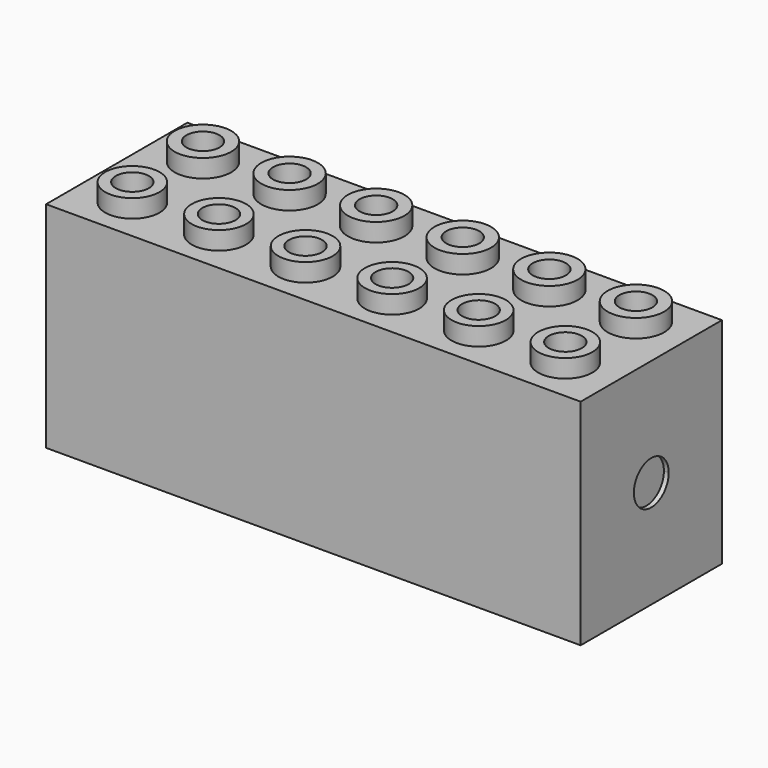
from build123d import *

# Parameters (mm, degrees)
F1_DEPTH  = 19.2532
F4_DEPTH  = 1.6256
F7_DEPTH  = 0.4318
F9_DEPTH  = 19.2532
F10_DEPTH = 2.032


with BuildPart() as f1:
    # F0 (on Top) → F1 (new body)
    with BuildSketch(Plane.XY):
        Polygon((0, 7.9248), (0, 0), (47.9806, 0), (47.9806, 7.9248), (46.4566, 7.9248), (46.4566, 1.524), (1.524, 1.524), (1.524, 7.9248), align=None)
        Polygon((0, 15.8496), (0, 7.9248), (1.524, 7.9248), (1.524, 14.3256), (46.4566, 14.3256), (46.4566, 7.9248), (47.9806, 7.9248), (47.9806, 15.8496), align=None)
    extrude(amount=F1_DEPTH)



with BuildPart() as f1b:
    # F0 (on Top) → F1, piece 2 (new body)
    with BuildSketch(Plane.XY):
        with BuildLine():
            ThreePointArc((36.6014, 7.9248), (39.8399, 4.6863), (43.0784, 7.9248))
            Line((43.0784, 7.9248), (42.2148, 7.9248))
            ThreePointArc((42.2148, 7.9248), (39.8399, 5.5499), (37.465, 7.9248))
            Line((37.465, 7.9248), (36.6014, 7.9248))
        make_face()
        with BuildLine():
            Line((42.2148, 7.9248), (43.0784, 7.9248))
            ThreePointArc((43.0784, 7.9248), (39.8399, 11.1633), (36.6014, 7.9248))
            Line((36.6014, 7.9248), (37.465, 7.9248))
            ThreePointArc((37.465, 7.9248), (39.8399, 10.2997), (42.2148, 7.9248))
        make_face()
    extrude(amount=F1_DEPTH)


with BuildPart() as f4:
    # F3 (on face) → F4 (new body)
    with BuildSketch(Plane.XY.offset(19.2532)):
        with BuildLine():
            ThreePointArc((7.0104, 3.9624), (4.572, 6.4008), (2.1336, 3.9624))
            Line((2.1336, 3.9624), (3.0861, 3.9624))
            ThreePointArc((3.0861, 3.9624), (4.572, 5.4483), (6.0579, 3.9624))
            Line((6.0579, 3.9624), (7.0104, 3.9624))
        make_face()
        with BuildLine():
            Line((3.0861, 3.9624), (2.1336, 3.9624))
            ThreePointArc((2.1336, 3.9624), (4.572, 1.524), (7.0104, 3.9624))
            Line((7.0104, 3.9624), (6.0579, 3.9624))
            ThreePointArc((6.0579, 3.9624), (4.572, 2.4765), (3.0861, 3.9624))
        make_face()
    extrude(amount=F4_DEPTH)


with BuildPart() as f4b:
    # F3 (on face) → F4, piece 2 (new body)
    with BuildSketch(Plane.XY.offset(19.2532)):
        with BuildLine():
            ThreePointArc((17.6784, 3.9624), (20.1168, 1.524), (22.5552, 3.9624))
            Line((22.5552, 3.9624), (21.6027, 3.9624))
            ThreePointArc((21.6027, 3.9624), (20.1168, 2.4765), (18.6309, 3.9624))
            Line((18.6309, 3.9624), (17.6784, 3.9624))
        make_face()
        with BuildLine():
            Line((21.6027, 3.9624), (22.5552, 3.9624))
            ThreePointArc((22.5552, 3.9624), (20.1168, 6.4008), (17.6784, 3.9624))
            Line((17.6784, 3.9624), (18.6309, 3.9624))
            ThreePointArc((18.6309, 3.9624), (20.1168, 5.4483), (21.6027, 3.9624))
        make_face()
    extrude(amount=F4_DEPTH)


with BuildPart() as f4c:
    # F3 (on face) → F4, piece 3 (new body)
    with BuildSketch(Plane.XY.offset(19.2532)):
        with BuildLine():
            ThreePointArc((30.3276, 3.9624), (27.8892, 6.4008), (25.4508, 3.9624))
            Line((25.4508, 3.9624), (26.4033, 3.9624))
            ThreePointArc((26.4033, 3.9624), (27.8892, 5.4483), (29.3751, 3.9624))
            Line((29.3751, 3.9624), (30.3276, 3.9624))
        make_face()
        with BuildLine():
            Line((26.4033, 3.9624), (25.4508, 3.9624))
            ThreePointArc((25.4508, 3.9624), (27.8892, 1.524), (30.3276, 3.9624))
            Line((30.3276, 3.9624), (29.3751, 3.9624))
            ThreePointArc((29.3751, 3.9624), (27.8892, 2.4765), (26.4033, 3.9624))
        make_face()
    extrude(amount=F4_DEPTH)


with BuildPart() as f4d:
    # F3 (on face) → F4, piece 4 (new body)
    with BuildSketch(Plane.XY.offset(19.2532)):
        with BuildLine():
            ThreePointArc((40.9956, 3.9624), (43.434, 1.524), (45.8724, 3.9624))
            Line((45.8724, 3.9624), (44.9199, 3.9624))
            ThreePointArc((44.9199, 3.9624), (43.434, 2.4765), (41.9481, 3.9624))
            Line((41.9481, 3.9624), (40.9956, 3.9624))
        make_face()
        with BuildLine():
            Line((44.9199, 3.9624), (45.8724, 3.9624))
            ThreePointArc((45.8724, 3.9624), (43.434, 6.4008), (40.9956, 3.9624))
            Line((40.9956, 3.9624), (41.9481, 3.9624))
            ThreePointArc((41.9481, 3.9624), (43.434, 5.4483), (44.9199, 3.9624))
        make_face()
    extrude(amount=F4_DEPTH)


with BuildPart() as f4e:
    # F3 (on face) → F4, piece 5 (new body)
    with BuildSketch(Plane.XY.offset(19.2532)):
        with BuildLine():
            ThreePointArc((14.7828, 3.9624), (12.3444, 6.4008), (9.906, 3.9624))
            Line((9.906, 3.9624), (10.8585, 3.9624))
            ThreePointArc((10.8585, 3.9624), (12.3444, 5.4483), (13.8303, 3.9624))
            Line((13.8303, 3.9624), (14.7828, 3.9624))
        make_face()
        with BuildLine():
            Line((10.8585, 3.9624), (9.906, 3.9624))
            ThreePointArc((9.906, 3.9624), (12.3444, 1.524), (14.7828, 3.9624))
            Line((14.7828, 3.9624), (13.8303, 3.9624))
            ThreePointArc((13.8303, 3.9624), (12.3444, 2.4765), (10.8585, 3.9624))
        make_face()
    extrude(amount=F4_DEPTH)


with BuildPart() as f4f:
    # F3 (on face) → F4, piece 6 (new body)
    with BuildSketch(Plane.XY.offset(19.2532)):
        with BuildLine():
            ThreePointArc((38.1, 3.9624), (35.6616, 6.4008), (33.2232, 3.9624))
            Line((33.2232, 3.9624), (34.1757, 3.9624))
            ThreePointArc((34.1757, 3.9624), (35.6616, 5.4483), (37.1475, 3.9624))
            Line((37.1475, 3.9624), (38.1, 3.9624))
        make_face()
        with BuildLine():
            Line((34.1757, 3.9624), (33.2232, 3.9624))
            ThreePointArc((33.2232, 3.9624), (35.6616, 1.524), (38.1, 3.9624))
            Line((38.1, 3.9624), (37.1475, 3.9624))
            ThreePointArc((37.1475, 3.9624), (35.6616, 2.4765), (34.1757, 3.9624))
        make_face()
    extrude(amount=F4_DEPTH)


with BuildPart() as f1_1:
    add(f1.part)

    add(f1b.part)  # F4#7 merges F1b
    # F3 (on face) → F4, piece 7 (join)
    with BuildSketch(Plane.XY.offset(19.2532)):
        with BuildLine():
            ThreePointArc((7.1105154008, 11.8872), (4.572, 14.4257154008), (2.0334845992, 11.8872))
            Line((2.0334845992, 11.8872), (3.0861, 11.8872))
            ThreePointArc((3.0861, 11.8872), (4.572, 13.3731), (6.0579, 11.8872))
            Line((6.0579, 11.8872), (7.1105154008, 11.8872))
        make_face()
        with BuildLine():
            Line((3.0861, 11.8872), (2.0334845992, 11.8872))
            ThreePointArc((2.0334845992, 11.8872), (4.572, 9.3486845992), (7.1105154008, 11.8872))
            Line((7.1105154008, 11.8872), (6.0579, 11.8872))
            ThreePointArc((6.0579, 11.8872), (4.572, 10.4013), (3.0861, 11.8872))
        make_face()
        with BuildLine():
            ThreePointArc((40.8954845992, 11.8872), (43.434, 9.3486845992), (45.9725154008, 11.8872))
            Line((45.9725154008, 11.8872), (44.9199, 11.8872))
            ThreePointArc((44.9199, 11.8872), (43.434, 10.4013), (41.9481, 11.8872))
            Line((41.9481, 11.8872), (40.8954845992, 11.8872))
        make_face()
        with BuildLine():
            Line((44.9199, 11.8872), (45.9725154008, 11.8872))
            ThreePointArc((45.9725154008, 11.8872), (43.434, 14.4257154008), (40.8954845992, 11.8872))
            Line((40.8954845992, 11.8872), (41.9481, 11.8872))
            ThreePointArc((41.9481, 11.8872), (43.434, 13.3731), (44.9199, 11.8872))
        make_face()
        with BuildLine():
            ThreePointArc((14.8829154008, 11.8872), (12.3444, 14.4257154008), (9.8058845992, 11.8872))
            Line((9.8058845992, 11.8872), (10.8585, 11.8872))
            ThreePointArc((10.8585, 11.8872), (12.3444, 13.3731), (13.8303, 11.8872))
            Line((13.8303, 11.8872), (14.8829154008, 11.8872))
        make_face()
        with BuildLine():
            Line((10.8585, 11.8872), (9.8058845992, 11.8872))
            ThreePointArc((9.8058845992, 11.8872), (12.3444, 9.3486845992), (14.8829154008, 11.8872))
            Line((14.8829154008, 11.8872), (13.8303, 11.8872))
            ThreePointArc((13.8303, 11.8872), (12.3444, 10.4013), (10.8585, 11.8872))
        make_face()
        with BuildLine():
            ThreePointArc((33.1230845992, 11.8872), (35.6616, 9.3486845992), (38.2001154008, 11.8872))
            Line((38.2001154008, 11.8872), (37.1475, 11.8872))
            ThreePointArc((37.1475, 11.8872), (35.6616, 10.4013), (34.1757, 11.8872))
            Line((34.1757, 11.8872), (33.1230845992, 11.8872))
        make_face()
        with BuildLine():
            Line((37.1475, 11.8872), (38.2001154008, 11.8872))
            ThreePointArc((38.2001154008, 11.8872), (35.6616, 14.4257154008), (33.1230845992, 11.8872))
            Line((33.1230845992, 11.8872), (34.1757, 11.8872))
            ThreePointArc((34.1757, 11.8872), (35.6616, 13.3731), (37.1475, 11.8872))
        make_face()
        with BuildLine():
            ThreePointArc((22.6553154008, 11.8872), (20.1168, 14.4257154008), (17.5782845992, 11.8872))
            Line((17.5782845992, 11.8872), (18.6309, 11.8872))
            ThreePointArc((18.6309, 11.8872), (20.1168, 13.3731), (21.6027, 11.8872))
            Line((21.6027, 11.8872), (22.6553154008, 11.8872))
        make_face()
        with BuildLine():
            Line((18.6309, 11.8872), (17.5782845992, 11.8872))
            ThreePointArc((17.5782845992, 11.8872), (20.1168, 9.3486845992), (22.6553154008, 11.8872))
            Line((22.6553154008, 11.8872), (21.6027, 11.8872))
            ThreePointArc((21.6027, 11.8872), (20.1168, 10.4013), (18.6309, 11.8872))
        make_face()
        with BuildLine():
            ThreePointArc((25.3506845992, 11.8872), (27.8892, 9.3486845992), (30.4277154008, 11.8872))
            Line((30.4277154008, 11.8872), (29.3751, 11.8872))
            ThreePointArc((29.3751, 11.8872), (27.8892, 10.4013), (26.4033, 11.8872))
            Line((26.4033, 11.8872), (25.3506845992, 11.8872))
        make_face()
        with BuildLine():
            Line((29.3751, 11.8872), (30.4277154008, 11.8872))
            ThreePointArc((30.4277154008, 11.8872), (27.8892, 14.4257154008), (25.3506845992, 11.8872))
            Line((25.3506845992, 11.8872), (26.4033, 11.8872))
            ThreePointArc((26.4033, 11.8872), (27.8892, 13.3731), (29.3751, 11.8872))
        make_face()
    extrude(amount=F4_DEPTH)

    # F6 (on offset) → F7 (cut)
    with BuildSketch(Plane.YZ.offset(47.9806)):
        with BuildLine():
            ThreePointArc((9.1678369266, 11.1365711385), (6.4148288615, 10.8696369266), (6.6817630734, 8.1166288615))
            Line((6.6817630734, 8.1166288615), (9.1678369266, 11.1365711385))
        make_face()
        with BuildLine():
            Line((9.1678369266, 11.1365711385), (6.6817630734, 8.1166288615))
            ThreePointArc((6.6817630734, 8.1166288615), (8.7596718521, 7.8579444002), (9.8806, 9.6266))
            ThreePointArc((9.8806, 9.6266), (9.6934555998, 10.4614718521), (9.1678369266, 11.1365711385))
        make_face()
    extrude(amount=-F7_DEPTH, mode=Mode.SUBTRACT)

    # F0 (on Top) → F9 (join)
    with BuildSketch(Plane.XY):
        with BuildLine():
            Line((4.9022, 7.9248), (1.524, 7.9248))
            Line((1.524, 7.9248), (1.524, 1.524))
            Line((1.524, 1.524), (46.4566, 1.524))
            Line((46.4566, 1.524), (46.4566, 7.9248))
            Line((46.4566, 7.9248), (43.0784, 7.9248))
            ThreePointArc((43.0784, 7.9248), (39.8399, 4.6863), (36.6014, 7.9248))
            Line((36.6014, 7.9248), (35.1536, 7.9248))
            ThreePointArc((35.1536, 7.9248), (31.9151, 4.6863), (28.6766, 7.9248))
            Line((28.6766, 7.9248), (27.2288, 7.9248))
            ThreePointArc((27.2288, 7.9248), (23.9903, 4.6863), (20.7518, 7.9248))
            Line((20.7518, 7.9248), (19.304, 7.9248))
            ThreePointArc((19.304, 7.9248), (16.0655, 4.6863), (12.827, 7.9248))
            Line((12.827, 7.9248), (11.3792, 7.9248))
            ThreePointArc((11.3792, 7.9248), (8.1407, 4.6863), (4.9022, 7.9248))
        make_face()
        with BuildLine():
            Line((1.524, 14.3256), (1.524, 7.9248))
            Line((1.524, 7.9248), (4.9022, 7.9248))
            ThreePointArc((4.9022, 7.9248), (8.1407, 11.1633), (11.3792, 7.9248))
            Line((11.3792, 7.9248), (12.827, 7.9248))
            ThreePointArc((12.827, 7.9248), (16.0655, 11.1633), (19.304, 7.9248))
            Line((19.304, 7.9248), (20.7518, 7.9248))
            ThreePointArc((20.7518, 7.9248), (23.9903, 11.1633), (27.2288, 7.9248))
            Line((27.2288, 7.9248), (28.6766, 7.9248))
            ThreePointArc((28.6766, 7.9248), (31.9151, 11.1633), (35.1536, 7.9248))
            Line((35.1536, 7.9248), (36.6014, 7.9248))
            ThreePointArc((36.6014, 7.9248), (39.8399, 11.1633), (43.0784, 7.9248))
            Line((43.0784, 7.9248), (46.4566, 7.9248))
            Line((46.4566, 7.9248), (46.4566, 14.3256))
            Line((46.4566, 14.3256), (1.524, 14.3256))
        make_face()
        with BuildLine():
            Line((8.1407, 7.9248), (5.7658, 7.9248))
            ThreePointArc((5.7658, 7.9248), (8.1407, 5.5499), (10.5156, 7.9248))
            Line((10.5156, 7.9248), (8.1407, 7.9248))
        make_face()
        with BuildLine():
            Line((16.0655, 7.9248), (13.6906, 7.9248))
            ThreePointArc((13.6906, 7.9248), (16.0655, 5.5499), (18.4404, 7.9248))
            Line((18.4404, 7.9248), (16.0655, 7.9248))
        make_face()
        with BuildLine():
            ThreePointArc((18.4404, 7.9248), (16.0655, 10.2997), (13.6906, 7.9248))
            Line((13.6906, 7.9248), (16.0655, 7.9248))
            Line((16.0655, 7.9248), (18.4404, 7.9248))
        make_face()
        with BuildLine():
            Line((23.9903, 7.9248), (21.6154, 7.9248))
            ThreePointArc((21.6154, 7.9248), (23.9903, 5.5499), (26.3652, 7.9248))
            Line((26.3652, 7.9248), (23.9903, 7.9248))
        make_face()
        with BuildLine():
            ThreePointArc((26.3652, 7.9248), (23.9903, 10.2997), (21.6154, 7.9248))
            Line((21.6154, 7.9248), (23.9903, 7.9248))
            Line((23.9903, 7.9248), (26.3652, 7.9248))
        make_face()
        with BuildLine():
            ThreePointArc((29.5402, 7.9248), (31.9151, 5.5499), (34.29, 7.9248))
            Line((34.29, 7.9248), (31.9151, 7.9248))
            Line((31.9151, 7.9248), (29.5402, 7.9248))
        make_face()
        with BuildLine():
            Line((31.9151, 7.9248), (34.29, 7.9248))
            ThreePointArc((34.29, 7.9248), (31.9151, 10.2997), (29.5402, 7.9248))
            Line((29.5402, 7.9248), (31.9151, 7.9248))
        make_face()
        with BuildLine():
            Line((5.7658, 7.9248), (4.9022, 7.9248))
            ThreePointArc((4.9022, 7.9248), (8.1407, 4.6863), (11.3792, 7.9248))
            Line((11.3792, 7.9248), (10.5156, 7.9248))
            ThreePointArc((10.5156, 7.9248), (8.1407, 5.5499), (5.7658, 7.9248))
        make_face()
        with BuildLine():
            Line((13.6906, 7.9248), (12.827, 7.9248))
            ThreePointArc((12.827, 7.9248), (16.0655, 4.6863), (19.304, 7.9248))
            Line((19.304, 7.9248), (18.4404, 7.9248))
            ThreePointArc((18.4404, 7.9248), (16.0655, 5.5499), (13.6906, 7.9248))
        make_face()
        with BuildLine():
            ThreePointArc((19.304, 7.9248), (16.0655, 11.1633), (12.827, 7.9248))
            Line((12.827, 7.9248), (13.6906, 7.9248))
            ThreePointArc((13.6906, 7.9248), (16.0655, 10.2997), (18.4404, 7.9248))
            Line((18.4404, 7.9248), (19.304, 7.9248))
        make_face()
        with BuildLine():
            Line((21.6154, 7.9248), (20.7518, 7.9248))
            ThreePointArc((20.7518, 7.9248), (23.9903, 4.6863), (27.2288, 7.9248))
            Line((27.2288, 7.9248), (26.3652, 7.9248))
            ThreePointArc((26.3652, 7.9248), (23.9903, 5.5499), (21.6154, 7.9248))
        make_face()
        with BuildLine():
            ThreePointArc((27.2288, 7.9248), (23.9903, 11.1633), (20.7518, 7.9248))
            Line((20.7518, 7.9248), (21.6154, 7.9248))
            ThreePointArc((21.6154, 7.9248), (23.9903, 10.2997), (26.3652, 7.9248))
            Line((26.3652, 7.9248), (27.2288, 7.9248))
        make_face()
        with BuildLine():
            ThreePointArc((28.6766, 7.9248), (31.9151, 4.6863), (35.1536, 7.9248))
            Line((35.1536, 7.9248), (34.29, 7.9248))
            ThreePointArc((34.29, 7.9248), (31.9151, 5.5499), (29.5402, 7.9248))
            Line((29.5402, 7.9248), (28.6766, 7.9248))
        make_face()
        with BuildLine():
            Line((34.29, 7.9248), (35.1536, 7.9248))
            ThreePointArc((35.1536, 7.9248), (31.9151, 11.1633), (28.6766, 7.9248))
            Line((28.6766, 7.9248), (29.5402, 7.9248))
            ThreePointArc((29.5402, 7.9248), (31.9151, 10.2997), (34.29, 7.9248))
        make_face()
        with BuildLine():
            ThreePointArc((37.465, 7.9248), (39.8399, 5.5499), (42.2148, 7.9248))
            Line((42.2148, 7.9248), (39.8399, 7.9248))
            Line((39.8399, 7.9248), (37.465, 7.9248))
        make_face()
        with BuildLine():
            Line((39.8399, 7.9248), (42.2148, 7.9248))
            ThreePointArc((42.2148, 7.9248), (39.8399, 10.2997), (37.465, 7.9248))
            Line((37.465, 7.9248), (39.8399, 7.9248))
        make_face()
        with BuildLine():
            ThreePointArc((11.3792, 7.9248), (8.1407, 11.1633), (4.9022, 7.9248))
            Line((4.9022, 7.9248), (5.7658, 7.9248))
            ThreePointArc((5.7658, 7.9248), (8.1407, 10.2997), (10.5156, 7.9248))
            Line((10.5156, 7.9248), (11.3792, 7.9248))
        make_face()
        with BuildLine():
            ThreePointArc((10.5156, 7.9248), (8.1407, 10.2997), (5.7658, 7.9248))
            Line((5.7658, 7.9248), (8.1407, 7.9248))
            Line((8.1407, 7.9248), (10.5156, 7.9248))
        make_face()
    extrude(amount=F9_DEPTH)

    # F0 (on Top) → F10 (cut)
    with BuildSketch(Plane.XY):
        with BuildLine():
            Line((1.524, 14.3256), (1.524, 7.9248))
            Line((1.524, 7.9248), (4.9022, 7.9248))
            ThreePointArc((4.9022, 7.9248), (8.1407, 11.1633), (11.3792, 7.9248))
            Line((11.3792, 7.9248), (12.827, 7.9248))
            ThreePointArc((12.827, 7.9248), (16.0655, 11.1633), (19.304, 7.9248))
            Line((19.304, 7.9248), (20.7518, 7.9248))
            ThreePointArc((20.7518, 7.9248), (23.9903, 11.1633), (27.2288, 7.9248))
            Line((27.2288, 7.9248), (28.6766, 7.9248))
            ThreePointArc((28.6766, 7.9248), (31.9151, 11.1633), (35.1536, 7.9248))
            Line((35.1536, 7.9248), (36.6014, 7.9248))
            ThreePointArc((36.6014, 7.9248), (39.8399, 11.1633), (43.0784, 7.9248))
            Line((43.0784, 7.9248), (46.4566, 7.9248))
            Line((46.4566, 7.9248), (46.4566, 14.3256))
            Line((46.4566, 14.3256), (1.524, 14.3256))
        make_face()
        with BuildLine():
            Line((4.9022, 7.9248), (1.524, 7.9248))
            Line((1.524, 7.9248), (1.524, 1.524))
            Line((1.524, 1.524), (46.4566, 1.524))
            Line((46.4566, 1.524), (46.4566, 7.9248))
            Line((46.4566, 7.9248), (43.0784, 7.9248))
            ThreePointArc((43.0784, 7.9248), (39.8399, 4.6863), (36.6014, 7.9248))
            Line((36.6014, 7.9248), (35.1536, 7.9248))
            ThreePointArc((35.1536, 7.9248), (31.9151, 4.6863), (28.6766, 7.9248))
            Line((28.6766, 7.9248), (27.2288, 7.9248))
            ThreePointArc((27.2288, 7.9248), (23.9903, 4.6863), (20.7518, 7.9248))
            Line((20.7518, 7.9248), (19.304, 7.9248))
            ThreePointArc((19.304, 7.9248), (16.0655, 4.6863), (12.827, 7.9248))
            Line((12.827, 7.9248), (11.3792, 7.9248))
            ThreePointArc((11.3792, 7.9248), (8.1407, 4.6863), (4.9022, 7.9248))
        make_face()
        with BuildLine():
            Line((16.0655, 7.9248), (13.6906, 7.9248))
            ThreePointArc((13.6906, 7.9248), (16.0655, 5.5499), (18.4404, 7.9248))
            Line((18.4404, 7.9248), (16.0655, 7.9248))
        make_face()
        with BuildLine():
            Line((8.1407, 7.9248), (5.7658, 7.9248))
            ThreePointArc((5.7658, 7.9248), (8.1407, 5.5499), (10.5156, 7.9248))
            Line((10.5156, 7.9248), (8.1407, 7.9248))
        make_face()
        with BuildLine():
            ThreePointArc((10.5156, 7.9248), (8.1407, 10.2997), (5.7658, 7.9248))
            Line((5.7658, 7.9248), (8.1407, 7.9248))
            Line((8.1407, 7.9248), (10.5156, 7.9248))
        make_face()
        with BuildLine():
            ThreePointArc((18.4404, 7.9248), (16.0655, 10.2997), (13.6906, 7.9248))
            Line((13.6906, 7.9248), (16.0655, 7.9248))
            Line((16.0655, 7.9248), (18.4404, 7.9248))
        make_face()
        with BuildLine():
            Line((23.9903, 7.9248), (21.6154, 7.9248))
            ThreePointArc((21.6154, 7.9248), (23.9903, 5.5499), (26.3652, 7.9248))
            Line((26.3652, 7.9248), (23.9903, 7.9248))
        make_face()
        with BuildLine():
            ThreePointArc((26.3652, 7.9248), (23.9903, 10.2997), (21.6154, 7.9248))
            Line((21.6154, 7.9248), (23.9903, 7.9248))
            Line((23.9903, 7.9248), (26.3652, 7.9248))
        make_face()
        with BuildLine():
            ThreePointArc((29.5402, 7.9248), (31.9151, 5.5499), (34.29, 7.9248))
            Line((34.29, 7.9248), (31.9151, 7.9248))
            Line((31.9151, 7.9248), (29.5402, 7.9248))
        make_face()
        with BuildLine():
            Line((31.9151, 7.9248), (34.29, 7.9248))
            ThreePointArc((34.29, 7.9248), (31.9151, 10.2997), (29.5402, 7.9248))
            Line((29.5402, 7.9248), (31.9151, 7.9248))
        make_face()
        with BuildLine():
            ThreePointArc((37.465, 7.9248), (39.8399, 5.5499), (42.2148, 7.9248))
            Line((42.2148, 7.9248), (39.8399, 7.9248))
            Line((39.8399, 7.9248), (37.465, 7.9248))
        make_face()
        with BuildLine():
            Line((39.8399, 7.9248), (42.2148, 7.9248))
            ThreePointArc((42.2148, 7.9248), (39.8399, 10.2997), (37.465, 7.9248))
            Line((37.465, 7.9248), (39.8399, 7.9248))
        make_face()
    extrude(amount=F10_DEPTH, mode=Mode.SUBTRACT)


solid = Compound([f4.part, f4b.part, f4c.part, f4d.part, f4e.part, f4f.part, f1_1.part])
